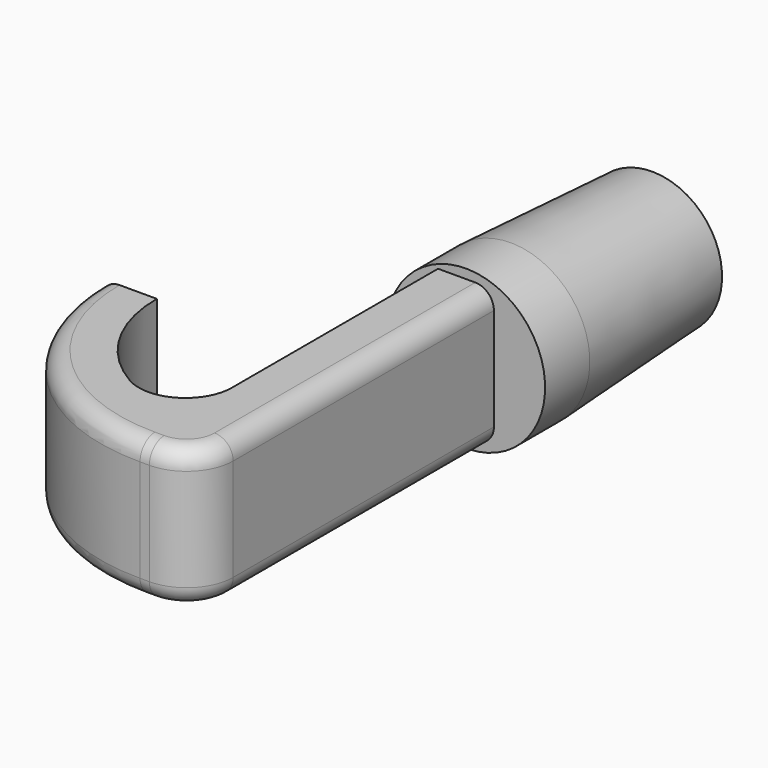
from build123d import *

# Parameters (mm, degrees)
F1_DEPTH    = 15
F2_R        = 8.5
F2_W        = 6
F2_H        = 15
F3_DEPTH    = 25
F4_SIZE2    = 19
F4_SIZE     = 1
F5_R        = 2
F6_R        = 5
F7_T1_DEPTH = 15
F7_T4_ANGLE = 90
F7_T6_ANGLE = 90


# Not quite as in the source:
# - a fillet or chamfer that OpenCascade refuses, or shapes differently, is made with other operations: its cross-section is extruded or revolved along the edge and cut away or added


with BuildPart() as f1:
    # F0 (on Top) → F1 (new body)
    with BuildSketch(Plane.XY):
        with BuildLine():
            ThreePointArc((-21, 0), (-14.8492424049, -14.8492424049), (0, -21))
            Line((0, -21), (0, -15))
            ThreePointArc((0, -15), (-10.6066017178, -10.6066017178), (-15, 0))
            Line((-15, 0), (-21, 0))
        make_face()
        Polygon((0, -15), (0, -21), (6, -21), (6, 19), (0, 19), (0, 0), align=None)
    extrude(amount=F1_DEPTH)

    # F2 (on face) → F3 (join)
    with BuildSketch(Plane(origin=(0, 19, 0), x_dir=(-1, 0, 0), z_dir=(0, 1, 0))):
        with Locations((-3, 7.5)):
            Circle(F2_R)
        with Locations((-3, 7.5)):
            Rectangle(F2_W, F2_H, mode=Mode.SUBTRACT)
        with Locations((-3, 7.5)):
            Rectangle(F2_W, F2_H)
    extrude(amount=F3_DEPTH)

    # F4
    f4_edges = [f1.edges().sort_by_distance(p)[0] for p in [
        (11.5, 44, 7.5),
    ]]
    f4_side = f1.faces().sort_by_distance((3, 44, 7.5))[0]
    chamfer(f4_edges, length=F4_SIZE, length2=F4_SIZE2, reference=f4_side)

    # F5
    f5_edges = [f1.edges().sort_by_distance(p)[0] for p in [
        (6, -1, 15),
        (-14.849242, -14.849242, 15),
        (3, -21, 0),
        (-14.849242, -14.849242, 0),
        (6, -1, 0),
    ]]
    fillet(f5_edges, radius=F5_R)

    # F6
    f6_edges = [f1.edges().sort_by_distance(p)[0] for p in [
        (0, -15, 7.5),
    ]]
    fillet(f6_edges, radius=F6_R)

    # F7: fillet of radius 5 on 1 edges, made by hand

    # F7_s2 → F7_t1 (cut)
    with BuildSketch(Plane.XY):
        with BuildLine():
            ThreePointArc((6, -16), (4.5355339059, -19.5355339059), (1, -21))
            Line((1, -21), (6, -21))
            Line((6, -21), (6, -16))
        make_face()
    extrude(amount=F7_T1_DEPTH, mode=Mode.SUBTRACT)

    # F7_s3 → F7_t4 (revolve, cut)
    with BuildSketch(Plane.XZ.offset(16)):
        with BuildLine():
            ThreePointArc((4, 0), (5.4142135624, 0.5857864376), (6, 2))
            Line((6, 2), (6, 0))
            Line((6, 0), (4, 0))
        make_face()
    revolve(axis=Axis((1, -16, 0), (0, 0, -1)), revolution_arc=F7_T4_ANGLE, mode=Mode.SUBTRACT)

    # F7_s5 → F7_t6 (revolve, cut)
    with BuildSketch(Plane.YZ.offset(1)):
        with BuildLine():
            ThreePointArc((-19, 15), (-20.4142135624, 14.4142135624), (-21, 13))
            Line((-21, 13), (-21, 15))
            Line((-21, 15), (-19, 15))
        make_face()
    revolve(axis=Axis((1, -16, 15), (0, 0, 1)), revolution_arc=F7_T6_ANGLE, mode=Mode.SUBTRACT)


solid = f1.part
